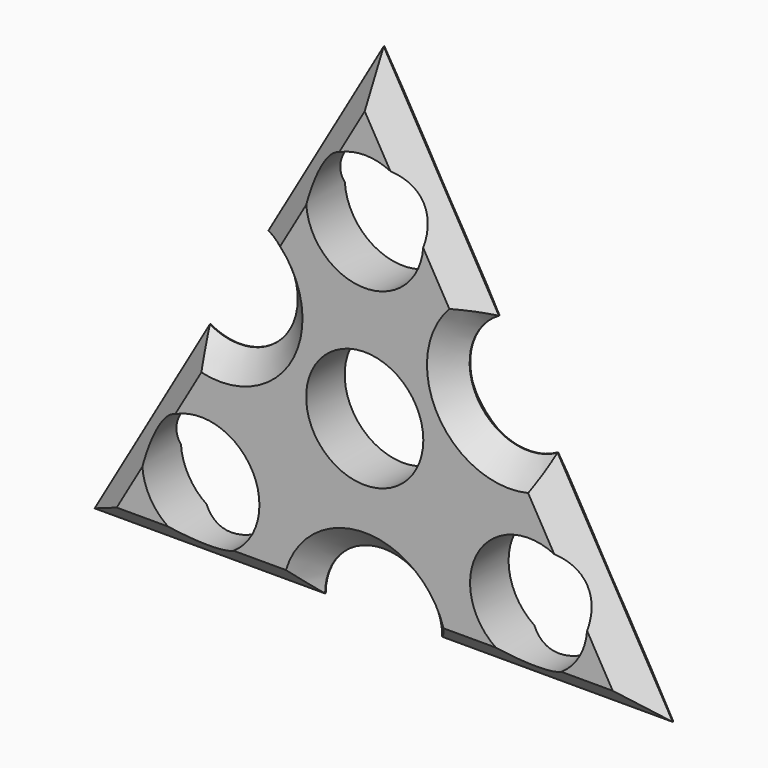
from build123d import *

# Parameters (mm, degrees)
F0_R         = 7.7216
F1_DEPTH     = 6.35
F2_T1_DEPTH  = 46.447303982
F2_T3_DEPTH  = 46.447303982
F2_T5_DEPTH  = 46.447303982
F2_T7_DEPTH  = 46.447303982
F2_T9_DEPTH  = 46.447303982
F2_T11_DEPTH = 46.447303982
F2_T14_ANGLE = 299.426156199
F2_T16_ANGLE = 299.426156199
F2_T18_ANGLE = 299.426156199
F2_T20_ANGLE = 299.426156199
F2_T22_ANGLE = 299.426156199
F2_T24_ANGLE = 299.426156199


# Not quite as in the source:
# - a fillet or chamfer that OpenCascade refuses, or shapes differently, is made with other operations: its cross-section is extruded or revolved along the edge and cut away or added


with BuildPart() as f1:
    # F0 (on Front) → F1 (new body)
    with BuildSketch(Plane.XZ):
        with BuildLine():
            Line((-22.9108, 2.227330358), (-38.1, -24.0811357684))
            Line((-38.1, -24.0811357684), (-7.7216, -24.0811357684))
            ThreePointArc((-7.7216, -24.0811357684), (0, -16.3595357684), (7.7216, -24.0811357684))
            Line((7.7216, -24.0811357684), (38.1, -24.0811357684))
            Line((38.1, -24.0811357684), (22.9108, 2.227330358))
            ThreePointArc((22.9108, 2.227330358), (12.3628982421, 5.0536321158), (15.1892, 15.6015338737))
            Line((15.1892, 15.6015338737), (0, 41.91))
            Line((0, 41.91), (-15.1892, 15.6015338737))
            ThreePointArc((-15.1892, 15.6015338737), (-12.3628982421, 12.7752321158), (-11.3284, 8.9144321158))
            ThreePointArc((-11.3284, 8.9144321158), (-15.1892, 2.227330358), (-22.9108, 2.227330358))
        make_face()
        with Locations((-21.6022160579, -14.5561357684)):
            Circle(F0_R, mode=Mode.SUBTRACT)
        with Locations((21.6022160579, -14.5561357684)):
            Circle(F0_R, mode=Mode.SUBTRACT)
        Circle(F0_R, mode=Mode.SUBTRACT)
        with Locations((0, 22.86)):
            Circle(F0_R, mode=Mode.SUBTRACT)
    extrude(amount=F1_DEPTH)

    # F2: chamfer of 3.1242 on 18 edges, made by hand

    # F2_s2 → F2_t1 (cut)
    with BuildSketch(Plane(origin=(-0.7460116682, 0, -1.2921301124), x_dir=(0, 1, 0), z_dir=(-0.5, 0, -0.8660254038))):
        Polygon((-6.35, -17.8308), (-3.2258, -20.955), (-6.35, -20.955), align=None)
        Polygon((-3.1242, -20.955), (0, -17.8308), (0, -20.955), align=None)
    extrude(amount=F2_T1_DEPTH, mode=Mode.SUBTRACT)

    # F2_s4 → F2_t3 (cut)
    with BuildSketch(Plane(origin=(22.1647883318, 0, 38.3905395297), x_dir=(0, 1, 0), z_dir=(-0.5, 0, -0.8660254038))):
        Polygon((-6.35, -17.8308), (-3.2258, -20.955), (-6.35, -20.955), align=None)
        Polygon((-3.1242, -20.955), (0, -17.8308), (0, -20.955), align=None)
    extrude(amount=F2_T3_DEPTH, mode=Mode.SUBTRACT)

    # F2_s6 → F2_t5 (cut)
    with BuildSketch(Plane(origin=(1.0588636592, 0, -1.834005656), x_dir=(0, 1, 0), z_dir=(-0.5, 0, 0.8660254038))):
        Polygon((-6.35, -17.8308), (-3.2258, -20.955), (-6.35, -20.955), align=None)
        Polygon((0, -17.8308), (-3.1242, -20.955), (0, -20.955), align=None)
    extrude(amount=F2_T5_DEPTH, mode=Mode.SUBTRACT)

    # F2_s8 → F2_t7 (cut)
    with BuildSketch(Plane(origin=(23.9696636592, 0, -41.5166752981), x_dir=(0, 1, 0), z_dir=(-0.5, 0, 0.8660254038))):
        Polygon((-6.35, -17.8308), (-3.2258, -20.955), (-6.35, -20.955), align=None)
        Polygon((0, -17.8308), (-3.1242, -20.955), (0, -20.955), align=None)
    extrude(amount=F2_T7_DEPTH, mode=Mode.SUBTRACT)

    # F2_s10 → F2_t9 (cut)
    with BuildSketch(Plane.YZ.offset(-0.312851991)):
        Polygon((-6.35, -20.9569357684), (-3.2258, -24.0811357684), (-6.35, -24.0811357684), align=None)
        Polygon((-3.1242, -24.0811357684), (0, -20.9569357684), (0, -24.0811357684), align=None)
    extrude(amount=F2_T9_DEPTH, mode=Mode.SUBTRACT)

    # F2_s12 → F2_t11 (cut)
    with BuildSketch(Plane.YZ.offset(-46.134451991)):
        Polygon((-6.35, -20.9569357684), (-3.2258, -24.0811357684), (-6.35, -24.0811357684), align=None)
        Polygon((-3.1242, -24.0811357684), (0, -20.9569357684), (0, -24.0811357684), align=None)
    extrude(amount=F2_T11_DEPTH, mode=Mode.SUBTRACT)

    # F2_s13 → F2_t14 (revolve, cut)
    with BuildSketch(Plane(origin=(-0.0451180595, 0, 9.0096042642), x_dir=(0, 1, 0), z_dir=(-0.0050077109, 0, 0.9999874613))):
        Polygon((-6.35, 29.8509202393), (-3.2258, 26.7267202393), (-6.35, 26.7267202393), align=None)
    revolve(axis=Axis((-19.05, -6.35, 8.9144321158), (0, -1, 0)), revolution_arc=F2_T14_ANGLE, mode=Mode.SUBTRACT)

    # F2_s15 → F2_t16 (revolve, cut)
    with BuildSketch(Plane(origin=(0.0451180595, 0, 9.0096042642), x_dir=(0, 1, 0), z_dir=(0.0050077109, 0, 0.9999874613))):
        Polygon((-3.2258, -26.7267202393), (-6.35, -29.8509202393), (-6.35, -26.7267202393), align=None)
    revolve(axis=Axis((19.05, -6.35, 8.9144321158), (0, 1, 0)), revolution_arc=F2_T16_ANGLE, mode=Mode.SUBTRACT)

    # F2_s17 → F2_t18 (revolve, cut)
    with BuildSketch(Plane(origin=(10.4872096098, 0, -6.1250197631), x_dir=(0, 1, 0), z_dir=(0.8635106895, 0, -0.5043305355))):
        Polygon((-6.35, -31.6401181517), (-3.2258, -28.5159181517), (-6.35, -28.5159181517), align=None)
    revolve(axis=Axis((0, -6.35, -24.0811357684), (0, 1, 0)), revolution_arc=F2_T18_ANGLE, mode=Mode.SUBTRACT)

    # F2_s19 → F2_t20 (revolve, cut)
    with BuildSketch(Plane(origin=(10.4872096098, 0, -6.1250197631), x_dir=(0, 1, 0), z_dir=(0.8635106895, 0, -0.5043305355))):
        Polygon((-3.1242, -28.5159181517), (0, -31.6401181517), (0, -28.5159181517), align=None)
    revolve(axis=Axis((0, 0, -24.0811357684), (0, 1, 0)), revolution_arc=F2_T20_ANGLE, mode=Mode.SUBTRACT)

    # F2_s21 → F2_t22 (revolve, cut)
    with BuildSketch(Plane(origin=(0.0451180595, 0, 9.0096042642), x_dir=(0, 1, 0), z_dir=(0.0050077109, 0, 0.9999874613))):
        Polygon((-3.1242, -26.7267202393), (0, -29.8509202393), (0, -26.7267202393), align=None)
    revolve(axis=Axis((19.05, 0, 8.9144321158), (0, 1, 0)), revolution_arc=F2_T22_ANGLE, mode=Mode.SUBTRACT)

    # F2_s23 → F2_t24 (revolve, cut)
    with BuildSketch(Plane(origin=(-10.5323276693, 0, -6.0107202694), x_dir=(0, 1, 0), z_dir=(-0.8685184004, 0, -0.4956569258))):
        Polygon((-3.1242, -24.9062127584), (0, -28.0304127584), (0, -24.9062127584), align=None)
    revolve(axis=Axis((-19.05, 0, 8.9144321158), (0, 1, 0)), revolution_arc=F2_T24_ANGLE, mode=Mode.SUBTRACT)


solid = f1.part
